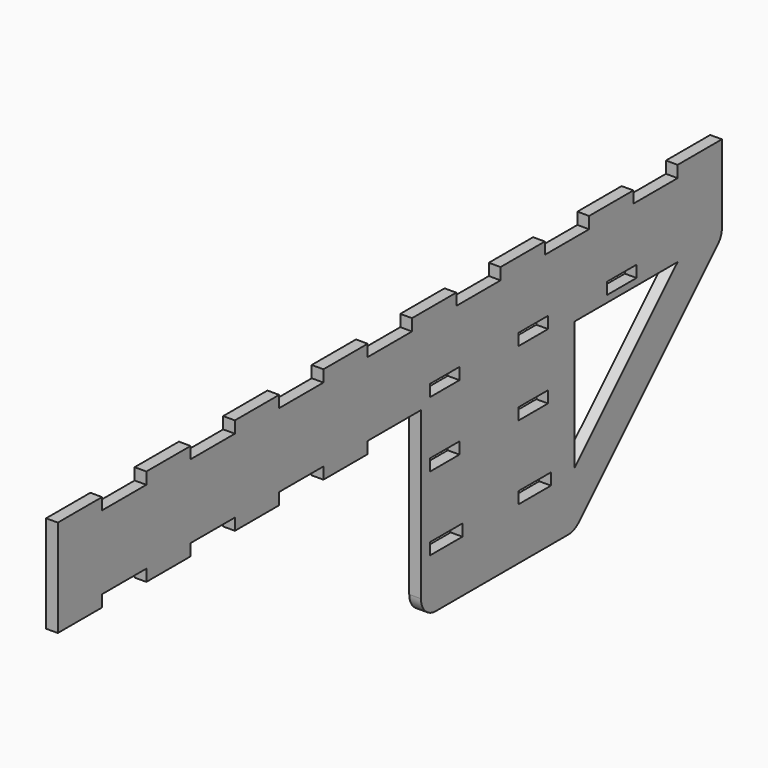
from build123d import *

# Parameters (mm, degrees)
F0_W     = 15
F0_H     = 3.175
F0_W_2   = 10
F0_W_3   = 11
F0_H_2   = 20
F1_DEPTH = 3.175
F2_R     = 5


# Not quite as in the source:
# - a feature names something its author has since deleted; it is built from what else it names


with BuildPart() as f1:
    # F0 (on Right) → F1 (new body)
    with BuildSketch(Plane.YZ):
        with Locations((-94.0358207209, -1.5875)):
            Rectangle(F0_W, F0_H)
        with Locations((-64.0358207209, -1.5875)):
            Rectangle(F0_W, F0_H)
        with Locations((-34.0358207209, -1.5875)):
            Rectangle(F0_W, F0_H)
        with Locations((-4.0358207209, -1.5875)):
            Rectangle(F0_W, F0_H)
        Polygon((-101.5358207209, 20), (-101.5358207209, 0), (-86.5358207209, 0), (-71.5358207209, 0), (-56.5358207209, 0), (-41.5358207209, 0), (-26.5358207209, 0), (-11.5358207209, 0), (3.4641792791, 0), (21.4992204921, 0), (38.0393435029, 0), (73.4641792791, 0), (108.4641792791, 0), (108.4641792791, 20), (93.4641792791, 20), (78.4641792791, 20), (63.4641792791, 20), (48.4641792791, 20), (33.4641792791, 20), (18.4641792791, 20), (3.4641792791, 20), (-11.5358207209, 20), (-26.5358207209, 20), (-41.5358207209, 20), (-56.5358207209, 20), (-71.5358207209, 20), (-86.5358207209, 20), align=None)
        with Locations((29.5455027372, 3.4310361944)):
            Rectangle(F0_W_2, F0_H, mode=Mode.SUBTRACT)
        with Locations((59.5455027372, 3.4310361944)):
            Rectangle(F0_W_2, F0_H, mode=Mode.SUBTRACT)
        with Locations((89.5455027372, 3.4310361944)):
            Rectangle(F0_W_2, F0_H, mode=Mode.SUBTRACT)
        Polygon((38.0393435029, 0), (21.4992204921, 0), (21.4992204921, -50), (73.4641792791, -50), (73.4641792791, -35), (73.4641792791, 0), align=None)
        with Locations((30.0455027372, -34.3287487835)):
            Rectangle(F0_W_3, F0_H, mode=Mode.SUBTRACT)
        with Locations((60.0455027372, -34.3287487835)):
            Rectangle(F0_W_3, F0_H, mode=Mode.SUBTRACT)
        with Locations((29.5455027372, -14.3287487835)):
            Rectangle(F0_W_2, F0_H, mode=Mode.SUBTRACT)
        with Locations((59.5455027372, -14.3287487835)):
            Rectangle(F0_W_2, F0_H, mode=Mode.SUBTRACT)
        with Locations((-94.0358207209, 21.5875)):
            Rectangle(F0_W, F0_H)
        with Locations((-64.0358207209, 21.5875)):
            Rectangle(F0_W, F0_H)
        with Locations((-34.0358207209, 21.5875)):
            Rectangle(F0_W, F0_H)
        with Locations((-4.0358207209, 21.5875)):
            Rectangle(F0_W, F0_H)
        with Locations((25.9641792791, 21.5875)):
            Rectangle(F0_W, F0_H)
        with Locations((55.9641792791, 21.5875)):
            Rectangle(F0_W, F0_H)
        with Locations((85.9641792791, 21.5875)):
            Rectangle(F0_W, F0_H)
        with Locations((115.9641792791, 21.5875)):
            Rectangle(F0_W, F0_H)
        with Locations((115.9641792791, 10)):
            Rectangle(F0_W, F0_H_2)
        Polygon((73.4641792791, -35), (73.4641792791, -50), (123.4641792791, 0), (108.4641792791, 0), align=None)
    extrude(amount=F1_DEPTH)

    # F2
    f2_edges = [f1.edges().sort_by_distance(p)[0] for p in [
        (1.5875, 123.464179, 0),
        (1.5875, 73.464179, -50),
        (1.5875, 21.49922, -50),
    ]]
    fillet(f2_edges, radius=F2_R)


solid = f1.part
